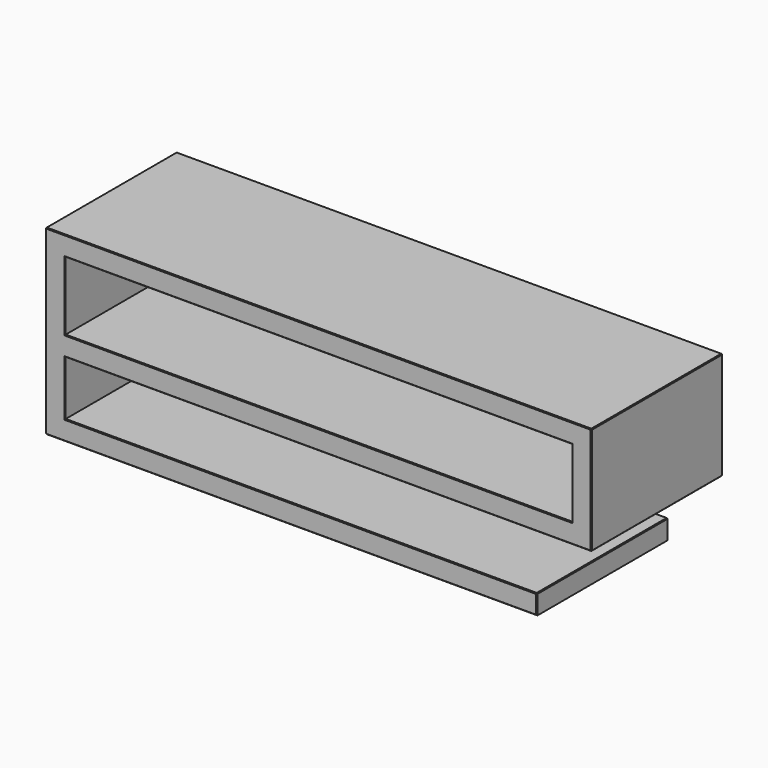
from build123d import *

# Parameters (mm, degrees)
F0_W     = 1392
F0_H     = 188
F1_DEPTH = 450
F2_SIZE  = 2


# Not quite as in the source:
# - a feature names something its author has since deleted; it is built from what else it names


with BuildPart() as f1:
    # F0 (on Front) → F1 (new body)
    with BuildSketch(Plane.XZ):
        Polygon((750, 250), (-750, 250), (-750, -250), (600, -250), (600, -196), (-696, -196), (-696, -46), (750, -46), align=None)
        with Locations((0, 102)):
            Rectangle(F0_W, F0_H, mode=Mode.SUBTRACT)
    extrude(amount=F1_DEPTH)

    # F2
    f2_edges = [f1.edges().sort_by_distance(p)[0] for p in [
        (-750, -225, 250),
        (-750, -225, -250),
        (-750, 0, 0),
        (-750, -450, 0),
        (750, -225, 250),
        (0, 0, 250),
        (0, -450, 250),
        (750, -225, -46),
        (750, 0, 102),
        (750, -450, 102),
        (-75, -450, -250),
        (600, -450, -223),
        (-48, -450, -196),
        (-696, -450, -121),
        (27, -450, -46),
        (-696, -450, 102),
        (0, -450, 196),
        (696, -450, 102),
        (0, -450, 8),
        (-75, 0, -250),
        (600, 0, -223),
        (-48, 0, -196),
        (-696, 0, -121),
        (27, 0, -46),
        (-696, 0, 102),
        (0, 0, 196),
        (696, 0, 102),
        (0, 0, 8),
        (600, -225, -196),
    ]]
    chamfer(f2_edges, length=F2_SIZE)


solid = f1.part
